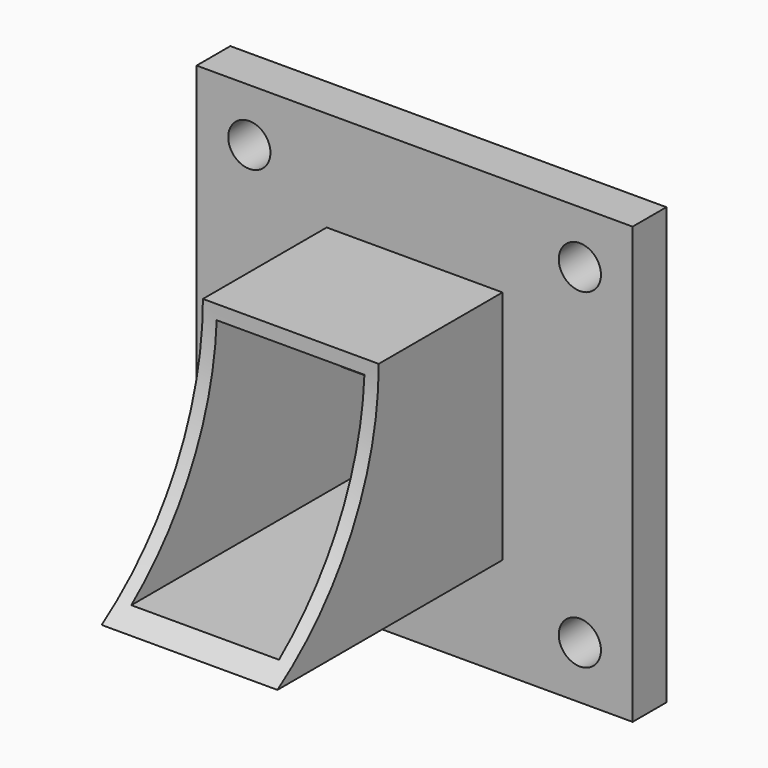
from build123d import *

# Parameters (mm, degrees)
F0_W         = 31
F0_H         = 31
F1_DEPTH     = 3
F2_R         = 1.5
F3_DEPTH     = 3
F4_W         = 12.5
F4_H         = 16.75
F5_DEPTH     = 20
F6_W         = 10.5
F6_H         = 14.75
F7_DEPTH     = 23
F8_R         = 20
F9_DEPTH     = 25
F10_W        = 12.5
F10_H        = 1
F11_DEPTH    = 3
F12_T1_DEPTH = 10.5
F13_W        = 12.5
F13_H        = 1
F14_DEPTH    = 3
F15_T1_DEPTH = 10.5


# Not quite as in the source:
# - a fillet or chamfer that OpenCascade refuses, or shapes differently, is made with other operations: its cross-section is extruded or revolved along the edge and cut away or added


with BuildPart() as f1:
    # F0 (on Front) → F1 (new body)
    with BuildSketch(Plane.XZ):
        Rectangle(F0_W, F0_H)
    extrude(amount=F1_DEPTH)

    # F2 (on face) → F3 (cut)
    with BuildSketch(Plane.XZ.offset(3)):
        with Locations((-11.75, -11.75)):
            Circle(F2_R)
        with Locations((-11.75, 11.75)):
            Circle(F2_R)
        with Locations((11.75, 11.75)):
            Circle(F2_R)
        with Locations((11.75, -11.75)):
            Circle(F2_R)
    extrude(amount=-F3_DEPTH, mode=Mode.SUBTRACT)

    # F4 (on face) → F5 (join)
    with BuildSketch(Plane.XZ.offset(3)):
        Rectangle(F4_W, F4_H)
    extrude(amount=F5_DEPTH)

    # F6 (on face) → F7 (cut)
    with BuildSketch(Plane.XZ.offset(23)):
        Rectangle(F6_W, F6_H)
    extrude(amount=-F7_DEPTH, mode=Mode.SUBTRACT)

    # F8 (on face) → F9 (cut)
    with BuildSketch(Plane.YZ.offset(6.25)):
        with Locations((-34, 8.3282930885)):
            Circle(F8_R)
    extrude(amount=-F9_DEPTH, mode=Mode.SUBTRACT)

    # F10 (on face) → F11 (join)
    with BuildSketch(Plane.XZ.offset(3)):
        with Locations((0, -0.5)):
            Rectangle(F10_W, F10_H)
    extrude(amount=-F11_DEPTH)

    # F12: fillet of radius 5 on 1 edges, made by hand

    # F12_s2 → F12_t1 (cut)
    with BuildSketch(Plane.YZ.offset(-5.25)):
        with BuildLine():
            ThreePointArc((0, -1), (-1.5811388301, -0.7434164903), (-3, 0))
            Line((-3, 0), (-3, -1))
            Line((-3, -1), (0, -1))
        make_face()
    extrude(amount=F12_T1_DEPTH, mode=Mode.SUBTRACT)

    # F13 (on face) → F14 (join)
    with BuildSketch(Plane.XZ.offset(3)):
        with Locations((0, 0.5)):
            Rectangle(F13_W, F13_H)
    extrude(amount=-F14_DEPTH)

    # F15: fillet of radius 5 on 1 edges, made by hand

    # F15_s2 → F15_t1 (cut)
    with BuildSketch(Plane.YZ.offset(-5.25)):
        with BuildLine():
            ThreePointArc((-3, 0), (-1.5811388301, 0.7434164903), (0, 1))
            Line((0, 1), (-3, 1))
            Line((-3, 1), (-3, 0))
        make_face()
    extrude(amount=F15_T1_DEPTH, mode=Mode.SUBTRACT)


solid = f1.part
